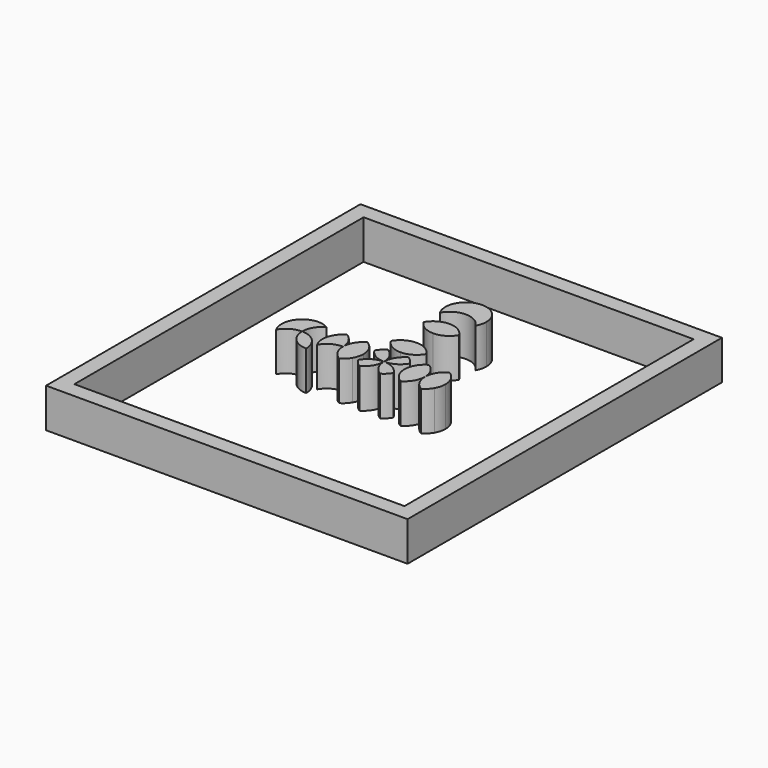
from build123d import *

# Parameters (mm, degrees)
F0_W     = 230
F0_H     = 250
F0_W_2   = 209.9999934435
F0_H_2   = 229.9999934435
F1_DEPTH = 25
F3_DEPTH = 25


with BuildPart() as f1:
    # F0 (on Top) → F1 (new body)
    with BuildSketch(Plane.XY):
        Rectangle(F0_W, F0_H)
        Rectangle(F0_W_2, F0_H_2, mode=Mode.SUBTRACT)
    extrude(amount=F1_DEPTH)


with BuildPart() as f3:
    # F2 (on Top) → F3 (new body)
    with BuildSketch(Plane.XY):
        with BuildLine():
            ThreePointArc((19.5404246493, 11.2816694314), (14.7722301011, 6.5134748831), (13.0269497662, 0))
            ThreePointArc((13.0269497662, 0), (13.4708323155, -3.3716226991), (14.7722301011, -6.5134748831))
            ThreePointArc((14.7722301011, -6.5134748831), (19.5404246493, -1.7452803349), (26.0538995325, 0))
            ThreePointArc((26.0538995325, 0), (24.3086191976, 6.5134748831), (19.5404246493, 11.2816694314))
        make_face()
        with BuildLine():
            ThreePointArc((26.0538995325, 0), (19.5404246493, -1.7452803349), (14.7722301011, -6.5134748831))
            ThreePointArc((14.7722301011, -6.5134748831), (16.8424550146, -9.2114445179), (19.5404246493, -11.2816694314))
            ThreePointArc((19.5404246493, -11.2816694314), (24.3086191976, -6.5134748831), (26.0538995325, 0))
        make_face()
    extrude(amount=F3_DEPTH)


with BuildPart() as f3b:
    # F2 (on Top) → F3, piece 2 (new body)
    with BuildSketch(Plane.XY):
        with BuildLine():
            ThreePointArc((0, 0), (6.5134748831, 1.7452803349), (11.2816694314, 6.5134748831))
            ThreePointArc((11.2816694314, 6.5134748831), (9.2114445179, 9.2114445179), (6.5134748831, 11.2816694314))
            ThreePointArc((6.5134748831, 11.2816694314), (1.7452803349, 6.5134748831), (0, 0))
        make_face()
    extrude(amount=F3_DEPTH)


with BuildPart() as f3c:
    # F2 (on Top) → F3, piece 3 (new body)
    with BuildSketch(Plane.XY):
        with BuildLine():
            ThreePointArc((6.5134748831, -11.2816694314), (9.2114445179, -9.2114445179), (11.2816694314, -6.5134748831))
            ThreePointArc((11.2816694314, -6.5134748831), (6.5134748831, -1.7452803349), (0, 0))
            ThreePointArc((0, 0), (1.7452803349, -6.5134748831), (6.5134748831, -11.2816694314))
        make_face()
    extrude(amount=F3_DEPTH)


with BuildPart() as f3d:
    # F2 (on Top) → F3, piece 4 (new body)
    with BuildSketch(Plane.XY):
        with BuildLine():
            ThreePointArc((-11.2816694314, 6.5134748831), (-6.5134748831, 1.7452803349), (0, 0))
            ThreePointArc((0, 0), (-1.7452803349, 6.5134748831), (-6.5134748831, 11.2816694314))
            ThreePointArc((-6.5134748831, 11.2816694314), (-9.2114445179, 9.2114445179), (-11.2816694314, 6.5134748831))
        make_face()
    extrude(amount=F3_DEPTH)


with BuildPart() as f3e:
    # F2 (on Top) → F3, piece 5 (new body)
    with BuildSketch(Plane.XY):
        with BuildLine():
            ThreePointArc((-6.5134748831, -11.2816694314), (-1.7452803349, -6.5134748831), (0, 0))
            ThreePointArc((0, 0), (-6.5134748831, -1.7452803349), (-11.2816694314, -6.5134748831))
            ThreePointArc((-11.2816694314, -6.5134748831), (-9.2114445179, -9.2114445179), (-6.5134748831, -11.2816694314))
        make_face()
    extrude(amount=F3_DEPTH)


with BuildPart() as f3f:
    # F2 (on Top) → F3, piece 6 (new body)
    with BuildSketch(Plane.XY):
        with BuildLine():
            ThreePointArc((37.3355689638, -6.5134748831), (32.5673744156, -1.7452803349), (26.0538995325, 0))
            ThreePointArc((26.0538995325, 0), (27.7991798673, -6.5134748831), (32.5673744156, -11.2816694314))
            ThreePointArc((32.5673744156, -11.2816694314), (35.2653440503, -9.2114445179), (37.3355689638, -6.5134748831))
        make_face()
        with BuildLine():
            ThreePointArc((32.5673744156, 11.2816694314), (27.7991798673, 6.5134748831), (26.0538995325, 0))
            ThreePointArc((26.0538995325, 0), (32.5673744156, -1.7452803349), (37.3355689638, -6.5134748831))
            ThreePointArc((37.3355689638, -6.5134748831), (38.6369667494, -3.3716226991), (39.0808492987, 0))
            ThreePointArc((39.0808492987, 0), (37.3355689638, 6.5134748831), (32.5673744156, 11.2816694314))
        make_face()
    extrude(amount=F3_DEPTH)


with BuildPart() as f3g:
    # F2 (on Top) → F3, piece 7 (new body)
    with BuildSketch(Plane.XY):
        with BuildLine():
            ThreePointArc((-11.2816694314, 19.5404246493), (-6.5134748831, 14.7722301011), (0, 13.0269497662))
            ThreePointArc((0, 13.0269497662), (6.5134748831, 14.7722301011), (11.2816694314, 19.5404246493))
            ThreePointArc((11.2816694314, 19.5404246493), (6.5134748329, 24.3086192266), (-1.16e-07, 26.0538995325))
            ThreePointArc((-1.16e-07, 26.0538995325), (-6.5134749333, 24.3086191686), (-11.2816694314, 19.5404246493))
        make_face()
    extrude(amount=F3_DEPTH)


with BuildPart() as f3h:
    # F2 (on Top) → F3, piece 8 (new body)
    with BuildSketch(Plane.XY):
        with BuildLine():
            ThreePointArc((-14.7722301011, -6.5134748831), (-13.4708323155, -3.3716226991), (-13.0269497662, 0))
            ThreePointArc((-13.0269497662, 0), (-14.7722301011, 6.5134748831), (-19.5404246493, 11.2816694314))
            ThreePointArc((-19.5404246493, 11.2816694314), (-24.3086191976, 6.5134748831), (-26.0538995325, 0))
            ThreePointArc((-26.0538995325, 0), (-19.5404246493, -1.7452803349), (-14.7722301011, -6.5134748831))
        make_face()
        with BuildLine():
            ThreePointArc((-26.0538995325, 0), (-24.3086191976, -6.5134748831), (-19.5404246493, -11.2816694314))
            ThreePointArc((-19.5404246493, -11.2816694314), (-16.8424550146, -9.2114445179), (-14.7722301011, -6.5134748831))
            ThreePointArc((-14.7722301011, -6.5134748831), (-19.5404246493, -1.7452803349), (-26.0538995325, 0))
        make_face()
    extrude(amount=F3_DEPTH)


with BuildPart() as f3i:
    # F2 (on Top) → F3, piece 9 (new body)
    with BuildSketch(Plane.XY):
        with BuildLine():
            ThreePointArc((-45.5943241818, -11.2816694314), (-42.4524719978, -12.583067217), (-39.0808492987, -13.0269497662))
            ThreePointArc((-39.0808492987, -13.0269497662), (-39.5247318479, -9.6553270671), (-40.8261296335, -6.5134748831))
            ThreePointArc((-40.8261296335, -6.5134748831), (-42.896354547, -9.2114445179), (-45.5943241818, -11.2816694314))
        make_face()
        with BuildLine():
            ThreePointArc((-52.1077990649, 0), (-50.3625187301, -6.5134748831), (-45.5943241818, -11.2816694314))
            ThreePointArc((-45.5943241818, -11.2816694314), (-42.896354547, -9.2114445179), (-40.8261296335, -6.5134748831))
            ThreePointArc((-40.8261296335, -6.5134748831), (-45.5943241818, -1.7452803349), (-52.1077990649, 0))
        make_face()
    extrude(amount=F3_DEPTH)


with BuildPart() as f3j:
    # F2 (on Top) → F3, piece 10 (new body)
    with BuildSketch(Plane.XY):
        with BuildLine():
            ThreePointArc((-37.3355689638, -6.5134748831), (-32.5673744156, -1.7452803349), (-26.0538995325, 0))
            ThreePointArc((-26.0538995325, 0), (-27.7991798673, 6.5134748831), (-32.5673744156, 11.2816694314))
            ThreePointArc((-32.5673744156, 11.2816694314), (-37.3355689638, 6.5134748831), (-39.0808492987, 0))
            ThreePointArc((-39.0808492987, 0), (-38.6369667494, -3.3716226991), (-37.3355689638, -6.5134748831))
        make_face()
    extrude(amount=F3_DEPTH)


with BuildPart() as f3k:
    # F2 (on Top) → F3, piece 11 (new body)
    with BuildSketch(Plane.XY):
        with BuildLine():
            ThreePointArc((-45.5943241818, 11.2816694314), (-61.3192435828, 9.2114445179), (-63.3894684963, -6.5134748831))
            ThreePointArc((-63.3894684963, -6.5134748831), (-58.621273948, -1.7452803349), (-52.1077990649, 0))
            ThreePointArc((-52.1077990649, 0), (-50.3625187301, 6.5134748831), (-45.5943241818, 11.2816694314))
        make_face()
    extrude(amount=F3_DEPTH)


with BuildPart() as f3l:
    # F2 (on Top) → F3, piece 12 (new body)
    with BuildSketch(Plane.XY):
        with BuildLine():
            ThreePointArc((-11.2816694314, 45.5943241818), (-6.513474888, 40.8261296364), (-1.14e-08, 39.0808492987))
            ThreePointArc((-1.14e-08, 39.0808492987), (6.5134748782, 40.8261296307), (11.2816694314, 45.5943241818))
            ThreePointArc((11.2816694314, 45.5943241818), (6.5134748436, 50.3625187529), (-9.13e-08, 52.1077990649))
            ThreePointArc((-9.13e-08, 52.1077990649), (-6.5134749226, 50.3625187072), (-11.2816694314, 45.5943241818))
        make_face()
    extrude(amount=F3_DEPTH)


with BuildPart() as f3m:
    # F2 (on Top) → F3, piece 13 (new body)
    with BuildSketch(Plane.XY):
        with BuildLine():
            ThreePointArc((13.0269497662, 65.1347488311), (-3.3716226991, 77.7178160481), (-11.2816694314, 58.621273948))
            ThreePointArc((-11.2816694314, 58.621273948), (0, 65.1347488311), (11.2816694314, 58.621273948))
            ThreePointArc((11.2816694314, 58.621273948), (12.583067217, 61.763126132), (13.0269497662, 65.1347488311))
        make_face()
    extrude(amount=F3_DEPTH)


solid = Compound([f1.part, f3.part, f3b.part, f3c.part, f3d.part, f3e.part, f3f.part, f3g.part, f3h.part, f3i.part, f3j.part, f3k.part, f3l.part, f3m.part])
